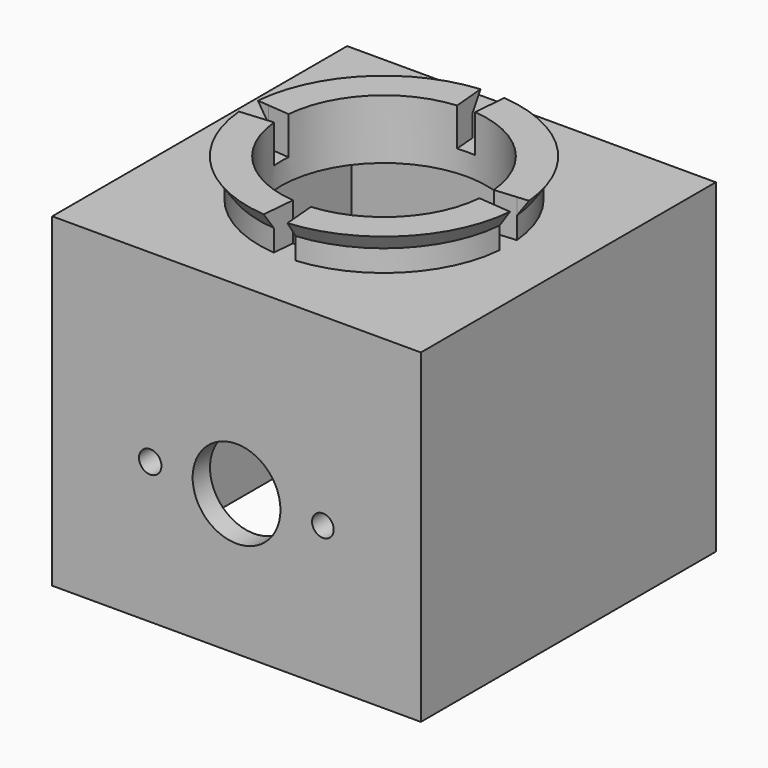
from build123d import *

# Parameters (mm, degrees)
F0_W      = 34
F0_H      = 34
F0_W_2    = 30
F0_H_2    = 30
F1_DEPTH  = 2
F2_DEPTH  = 28
F4_W      = 34
F4_H      = 34
F4_W_2    = 30
F4_H_2    = 30
F5_DEPTH  = 2
F9_DEPTH  = 3.5
F3_R      = 4.05
F3_R_2    = 1
F3_R_3    = 1.0373308001
F10_DEPTH = 2
F11_W     = 34
F11_H     = 34
F12_DEPTH = 2


with BuildPart() as f1:
    # F0 (on Top) → F1 (new body)
    with BuildSketch(Plane.XY):
        Rectangle(F0_W, F0_H)
        Rectangle(F0_W_2, F0_H_2, mode=Mode.SUBTRACT)
        Rectangle(F0_W_2, F0_H_2)
    extrude(amount=-F1_DEPTH)

    # F0 (on Top) → F2 (join)
    with BuildSketch(Plane.XY):
        Rectangle(F0_W, F0_H)
        Rectangle(F0_W_2, F0_H_2, mode=Mode.SUBTRACT)
    extrude(amount=F2_DEPTH)

    # F4 (on face) → F5 (join)
    with BuildSketch(Plane.XY.offset(28)):
        Rectangle(F4_W, F4_H)
        Rectangle(F4_W_2, F4_H_2, mode=Mode.SUBTRACT)
        Rectangle(F4_W_2, F4_H_2)
        with BuildLine():
            ThreePointArc((11.4562390281, 1.0022910416), (11.4890545482, 0.5016229547), (11.5, 0))
            ThreePointArc((11.5, 0), (11.4890545482, -0.5016229547), (11.4562390281, -1.0022910416))
            ThreePointArc((11.4562390281, -1.0022910416), (0, -11.5), (-11.4562390281, -1.0022910416))
            ThreePointArc((-11.4562390281, -1.0022910416), (-11.5, 0), (-11.4562390281, 1.0022910416))
            ThreePointArc((-11.4562390281, 1.0022910416), (0, 11.5), (11.4562390281, 1.0022910416))
        make_face(mode=Mode.SUBTRACT)
    extrude(amount=F5_DEPTH)

    # F6 (on Front) → F7 (revolve)
    with BuildSketch(Plane.XZ):
        Polygon((-11.5, 32), (-11.5, 30), (-9.5, 30), (-9.5, 33.5), (-12.5503113073, 33.5), align=None)
        Polygon((-9.5, 30), (-11.5, 30), (-11.5, 28), (-10.5, 28), (-9.5, 28), align=None)
    revolve(axis=Axis((0, 0, 27.9606003314), (0, 0, 1)))

    # F8 (on face) → F9 (cut)
    with BuildSketch(Plane.XY.offset(33.5)):
        with BuildLine():
            Line((9.4638496319, 0.8279795561), (0, 0))
            Line((0, 0), (9.4638496319, -0.8279795561))
            ThreePointArc((9.4638496319, -0.8279795561), (9.490958105, -0.41438418), (9.5, 0))
            ThreePointArc((9.5, 0), (9.490958105, 0.41438418), (9.4638496319, 0.8279795561))
        make_face()
        with BuildLine():
            Line((-9.4638496319, -0.8279795561), (0, 0))
            Line((0, 0), (-9.4638496319, 0.8279795561))
            ThreePointArc((-9.4638496319, 0.8279795561), (-9.5, 0), (-9.4638496319, -0.8279795561))
        make_face()
        with BuildLine():
            ThreePointArc((9.5, 0), (9.490958105, -0.41438418), (9.4638496319, -0.8279795561))
            Line((9.4638496319, -0.8279795561), (11.4562390281, -1.0022910416))
            Line((11.4562390281, -1.0022910416), (12.5025535837, -1.0938317037))
            ThreePointArc((12.5025535837, -1.0938317037), (12.5383661919, -0.5474368905), (12.5503113073, 0))
            ThreePointArc((12.5503113073, 0), (12.5383661919, 0.5474368905), (12.5025535837, 1.0938317037))
            Line((12.5025535837, 1.0938317037), (11.4562390281, 1.0022910416))
            Line((11.4562390281, 1.0022910416), (9.4638496319, 0.8279795561))
            ThreePointArc((9.4638496319, 0.8279795561), (9.490958105, 0.41438418), (9.5, 0))
        make_face()
        with BuildLine():
            Line((-11.4562390281, -1.0022910416), (-9.4638496319, -0.8279795561))
            ThreePointArc((-9.4638496319, -0.8279795561), (-9.5, 0), (-9.4638496319, 0.8279795561))
            Line((-9.4638496319, 0.8279795561), (-11.4562390281, 1.0022910416))
            Line((-11.4562390281, 1.0022910416), (-12.5025535837, 1.0938317037))
            ThreePointArc((-12.5025535837, 1.0938317037), (-12.5503113073, 0), (-12.5025535837, -1.0938317037))
            Line((-12.5025535837, -1.0938317037), (-11.4562390281, -1.0022910416))
        make_face()
        with BuildLine():
            Line((1.0938317037, -12.5025535837), (0.8279795561, -9.4638496319))
            ThreePointArc((0.8279795561, -9.4638496319), (0, -9.5), (-0.8279795561, -9.4638496319))
            Line((-0.8279795561, -9.4638496319), (-1.0938317037, -12.5025535837))
            ThreePointArc((-1.0938317037, -12.5025535837), (0, -12.5503113073), (1.0938317037, -12.5025535837))
        make_face()
        with BuildLine():
            Line((-1.0938317037, 12.5025535837), (-0.8279795561, 9.4638496319))
            ThreePointArc((-0.8279795561, 9.4638496319), (0, 9.5), (0.8279795561, 9.4638496319))
            Line((0.8279795561, 9.4638496319), (1.0938317037, 12.5025535837))
            ThreePointArc((1.0938317037, 12.5025535837), (0, 12.5503113073), (-1.0938317037, 12.5025535837))
        make_face()
    extrude(amount=-F9_DEPTH, mode=Mode.SUBTRACT)

    # F3 (on face) → F10 (cut, through all)
    with BuildSketch(Plane.XZ.offset(17)):
        with Locations((0, 13)):
            Circle(F3_R)
        with Locations((7.9639680702, 13)):
            Circle(F3_R_2)
        with Locations((-7.9639680702, 13)):
            Circle(F3_R_3)
    extrude(amount=-F10_DEPTH, mode=Mode.SUBTRACT)

    # F11 (on face) → F12 (cut)
    with BuildSketch(Plane(origin=(0, 0, -2), x_dir=(1, 0, 0), z_dir=(0, 0, -1))):
        Rectangle(F11_W, F11_H)
    extrude(amount=-F12_DEPTH, mode=Mode.SUBTRACT)


solid = f1.part
